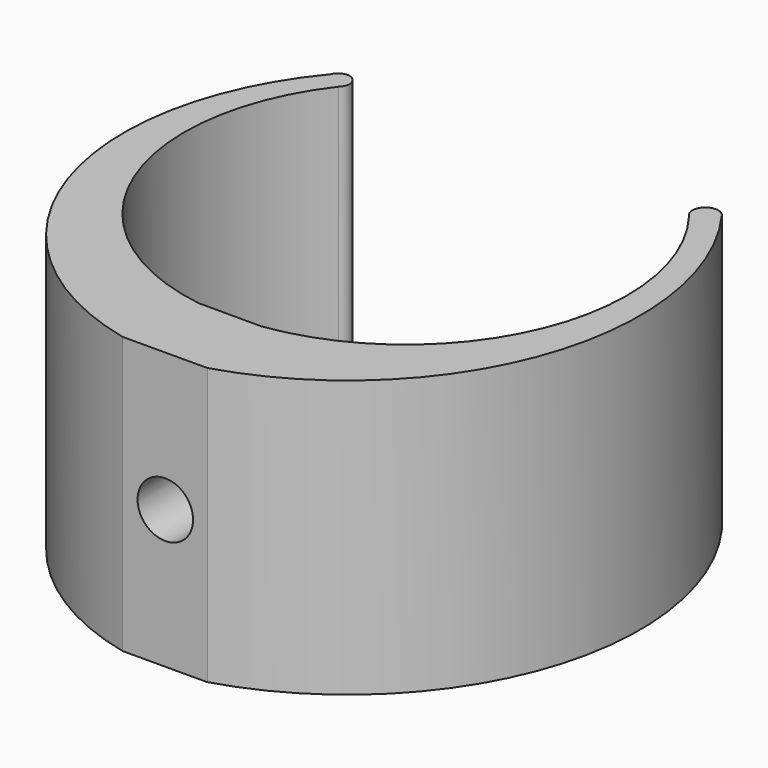
from build123d import *

# Parameters (mm, degrees)
F1_DEPTH = 15
F2_R     = 1.5
F3_DEPTH = 4.4278798556


# Not quite as in the source:
# - a feature names something its author has since deleted; it is built from what else it names


with BuildPart() as f1:
    # F0 (on Top) → F1 (new body)
    with BuildSketch(Plane.XY):
        with BuildLine():
            Line((1.7011785064, -11.877588293), (-1.7096480171, -11.877588293))
            ThreePointArc((-1.7096480171, -11.877588293), (-11.1202848878, -4.5099073176), (-9.5, 7.3314391493))
            ThreePointArc((-9.5, 7.3314391493), (-9.5385768198, 8.2900827327), (-10.4622412473, 8.0306030295))
            ThreePointArc((-10.4622412473, 8.0306030295), (-13.1913649606, -6.4201767786), (-2.3021989036, -16.3044681486))
            Line((-2.3021989036, -16.3044681486), (2.2770734892, -16.2874199147))
            ThreePointArc((2.2770734892, -16.2874199147), (12.7428435218, -6.1893456412), (10.5841437277, 8.1927078148))
            ThreePointArc((10.5841437277, 8.1927078148), (9.5441810303, 8.3863903947), (9.5, 7.3294687371))
            ThreePointArc((9.5, 7.3294687371), (11.1173000284, -4.5140615908), (1.7011785064, -11.877588293))
        make_face()
    extrude(amount=F1_DEPTH)

    # F2 (on face) → F3 (cut, through all)
    with BuildSketch(Plane(origin=(0, -11.877588293, 0), x_dir=(-1, 0, 0), z_dir=(0, 1, 0))):
        with Locations((0, 7.5)):
            Circle(F2_R)
    extrude(amount=-F3_DEPTH, mode=Mode.SUBTRACT)


solid = f1.part
